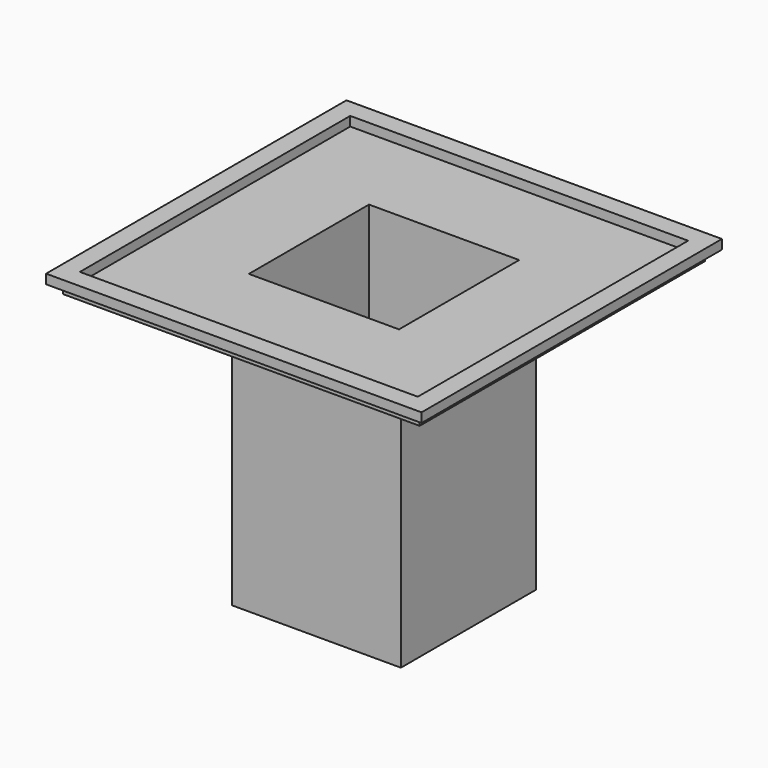
from build123d import *

# Parameters (mm, degrees)
F1_W        = 100
F1_H        = 100
F2_DEPTH    = 2.5
F4_W        = 95
F4_H        = 95
F5_DEPTH    = 2.5
F7_W        = 45
F7_H        = 45
F8_DEPTH    = 75
F9_T        = 2.5
F9_T3_DEPTH = 100
F9_T5_DEPTH = 100
F9_T7_DEPTH = 50
F9_T9_DEPTH = 50


# Not quite as in the source:
# - a shell that OpenCascade refuses in one call is made with other operations: the cavity is built on its own and cut out


with BuildPart() as f2:
    # F1 (on offset) → F2 (new body)
    with BuildSketch(Plane.XY.offset(80)):
        Rectangle(F1_W, F1_H)
    extrude(amount=-F2_DEPTH)

    # F4 (on offset) → F5 (join)
    with BuildSketch(Plane.XY.offset(77.5)):
        Rectangle(F4_W, F4_H)
    extrude(amount=-F5_DEPTH)

    # F7 (on offset) → F8 (join)
    with BuildSketch(Plane.XY.offset(75)):
        Rectangle(F7_W, F7_H)
    extrude(amount=-F8_DEPTH)

    # F9: shell of thickness 2.5, made by hand


with BuildPart() as f9_core1:
    # F9_t2: copy of F2
    add(f2.part)

    # the walls: a layer under each face that stays
    f9_faces = [f9_core1.faces().sort_by_distance(p)[0] for p in [
        (0, 50, 78.75),
        (50, 0, 78.75),
        (-50, 0, 78.75),
        (34.375, -48.7654320988, 77.5),
        (0, -50, 78.75),
        (-47.5, 0, 76.25),
        (0, -47.5, 76.25),
        (47.5, 0, 76.25),
        (0, 47.5, 76.25),
        (-31.6666666667, -31.6666666667, 75),
        (-22.5, 0, 37.5),
        (0, -22.5, 37.5),
        (22.5, 0, 37.5),
        (0, 22.5, 37.5),
        (0, 0, 0),
    ]]
    thicken(f9_faces, amount=-F9_T, mode=Mode.SUBTRACT)

    # F9_s4 → F9_t3 (cut)
    with BuildSketch(Plane.XZ.offset(-50)):
        Polygon((-47.525, 77.475), (-47.5, 80), (-45, 80), (-45, 77.5), align=None)
        Polygon((47.525, 77.475), (47.5, 80), (45, 80), (45, 77.5), align=None)
    extrude(amount=F9_T3_DEPTH, mode=Mode.SUBTRACT)

    # F9_s6 → F9_t5 (cut)
    with BuildSketch(Plane.YZ.offset(-50)):
        Polygon((-47.525, 77.475), (-47.5, 80), (-45, 80), (-45, 77.5), align=None)
        Polygon((47.525, 77.475), (47.5, 80), (45, 80), (45, 77.5), align=None)
    extrude(amount=F9_T5_DEPTH, mode=Mode.SUBTRACT)

    # F9_s8 → F9_t7 (cut)
    with BuildSketch(Plane.XZ.offset(-25)):
        Polygon((-22.525, 74.975), (-22.5, 77.5), (-20, 77.5), (-20, 75), align=None)
        Polygon((22.525, 74.975), (22.5, 77.5), (20, 77.5), (20, 75), align=None)
    extrude(amount=F9_T7_DEPTH, mode=Mode.SUBTRACT)

    # F9_s10 → F9_t9 (cut)
    with BuildSketch(Plane.YZ.offset(-25)):
        Polygon((-22.525, 74.975), (-22.5, 77.5), (-20, 77.5), (-20, 75), align=None)
        Polygon((22.525, 74.975), (22.5, 77.5), (20, 77.5), (20, 75), align=None)
    extrude(amount=F9_T9_DEPTH, mode=Mode.SUBTRACT)


with BuildPart() as f2_1:
    add(f2.part)

    # what is left inside the walls is the cavity
    f9_cavity = [f9_core1.part.solids().sort_by_distance(p)[0] for p in [
        (0, -15, 79.975),
    ]]
    add(f9_cavity, mode=Mode.SUBTRACT)


solid = f2_1.part
